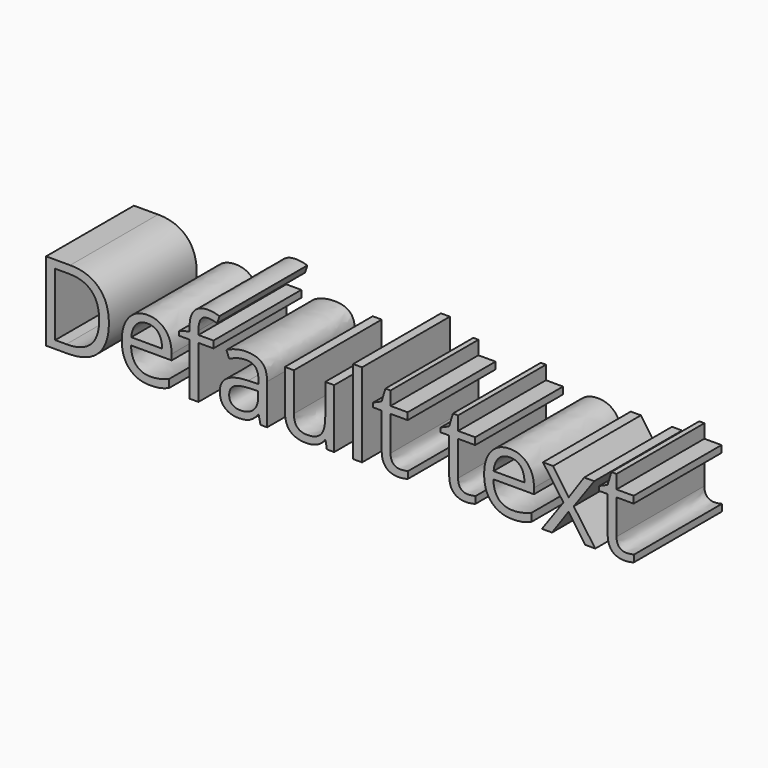
from build123d import *

# Parameters (mm, degrees)
F0_TEXT_SIZE = 25.4867494934
F1_DEPTH     = 25.4


# Not quite as in the source:
# - Text() gives the source's letters only with a copy of the font that has no kerning and outlines rounded to 1/6400 em; it was checked with that copy


with BuildPart() as f1:
    # F0 (on Front) → F1 (new body)
    with BuildSketch(Plane.XZ):
        with Locations((-110.6640920043, 30.4815247655)):
            Text('Default text', F0_TEXT_SIZE, font='Open Sans', text_align=(TextAlign.LEFT, TextAlign.BOTTOM))
    extrude(amount=F1_DEPTH)


solid = f1.part
